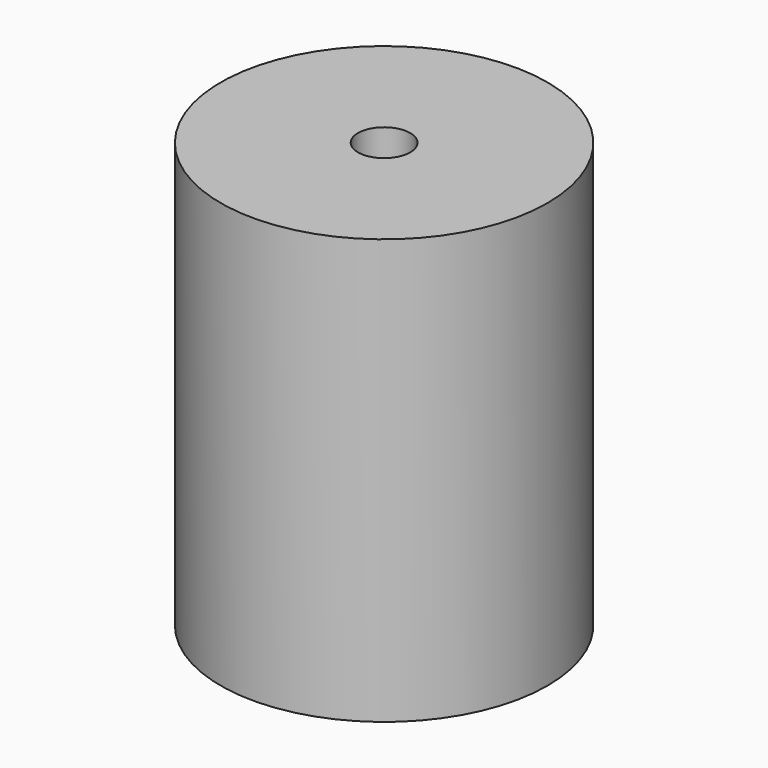
from build123d import *

# Parameters (mm, degrees)
F0_R     = 25
F1_DEPTH = 65
F2_R     = 4
F3_DEPTH = 65.001


# Not quite as in the source:
# - a feature names something its author has since deleted; it is built from what else it names


with BuildPart() as f1:
    # F0 (on Top) → F1 (new body)
    with BuildSketch(Plane.XY):
        Circle(F0_R)
    extrude(amount=F1_DEPTH)

    # F2 (on face) → F3 (cut, through all)
    with BuildSketch(Plane(origin=(0, 0, 0), x_dir=(1, 0, 0), z_dir=(0, 0, -1))):
        Circle(F2_R)
    extrude(amount=-F3_DEPTH, mode=Mode.SUBTRACT)


solid = f1.part
